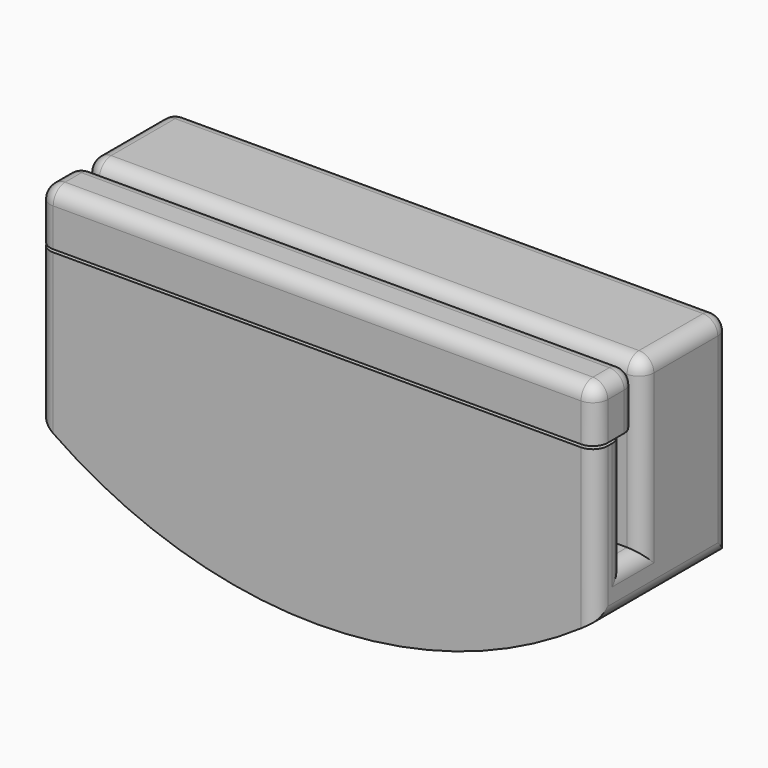
from build123d import *

# Parameters (mm, degrees)
F0_W     = 30
F0_H     = 5.9
F1_DEPTH = 16
F0_H_2   = 1.9
F2_DEPTH = 13
F0_H_3   = 1.2
F3_DEPTH = 7
F5_DEPTH = 9.001
F6_W     = 30
F6_H     = 1.9
F7_DEPTH = 2.85
F8_DEPTH = 0.8
F9_R     = 0.8
F9_2_R   = 0.8


with BuildPart() as f1:
    # F0 (on Top) → F1 (new body)
    with BuildSketch(Plane.XY):
        with Locations((0, 1.55)):
            Rectangle(F0_W, F0_H)
    extrude(amount=F1_DEPTH)



with BuildPart() as f2:
    # F0 (on Top) → F2 (new body)
    with BuildSketch(Plane.XY):
        with Locations((0, -3.55)):
            Rectangle(F0_W, F0_H_2)
    extrude(amount=F2_DEPTH)


with BuildPart() as f1_1:
    add(f1.part)

    add(f2.part)  # F3 merges F2
    # F0 (on Top) → F3 (join)
    with BuildSketch(Plane.XY):
        with Locations((0, -2)):
            Rectangle(F0_W, F0_H_3)
    extrude(amount=F3_DEPTH)

    # F4 (on face) → F5 (cut, through all)
    with BuildSketch(Plane.XZ.offset(4.5)):
        with BuildLine():
            ThreePointArc((0, 0), (-7.9056941504, 1.2829175487), (-15, 5))
            Line((-15, 5), (-15, 0))
            Line((-15, 0), (0, 0))
        make_face()
        with BuildLine():
            ThreePointArc((15, 5), (7.9056941504, 1.2829175487), (0, 0))
            Line((0, 0), (15, 0))
            Line((15, 0), (15, 5))
        make_face()
    extrude(amount=-F5_DEPTH, mode=Mode.SUBTRACT)

    # F9
    f9_edges = [f1_1.edges().sort_by_distance(p)[0] for p in [
        (-15, 0, 5),
        (15, 0, 5),
        (-15, -4.5, 9),
        (-15, -2.6, 10),
        (-15, -1.4, 11.5),
        (-15, -2, 7),
        (-15, 1.55, 16),
        (15, -1.4, 11.5),
        (15, -2.6, 10),
        (15, -4.5, 9),
        (15, -2, 7),
        (15, 1.55, 16),
        (0, -1.4, 16),
        (-15, 4.5, 10.5),
        (15, 4.5, 10.5),
        (0, 4.5, 16),
    ]]
    fillet(f9_edges, radius=F9_R)


with BuildPart() as f7:
    # F6 (on face) → F7 (new body, through all)
    with BuildSketch(Plane.XY.offset(16)):
        with Locations((0, -3.55)):
            Rectangle(F6_W, F6_H)
    extrude(amount=-F7_DEPTH)

    # F8 (add, through all): a face of the model
    f8_faces = [f7.faces().sort_by_distance(p)[0] for p in [
        (0, -2.6, 14.575),
    ]]
    extrude(f8_faces, amount=F8_DEPTH)

    # F9#2
    f9_2_edges = [f7.edges().sort_by_distance(p)[0] for p in [
        (-15, -4.5, 14.575),
        (-15, -3.15, 16),
        (0, -4.5, 16),
        (15, -4.5, 14.575),
        (15, -3.15, 16),
        (-15, -1.8, 14.575),
        (15, -1.8, 14.575),
        (0, -1.8, 16),
    ]]
    fillet(f9_2_edges, radius=F9_2_R)


solid = Compound([f1_1.part, f7.part])
